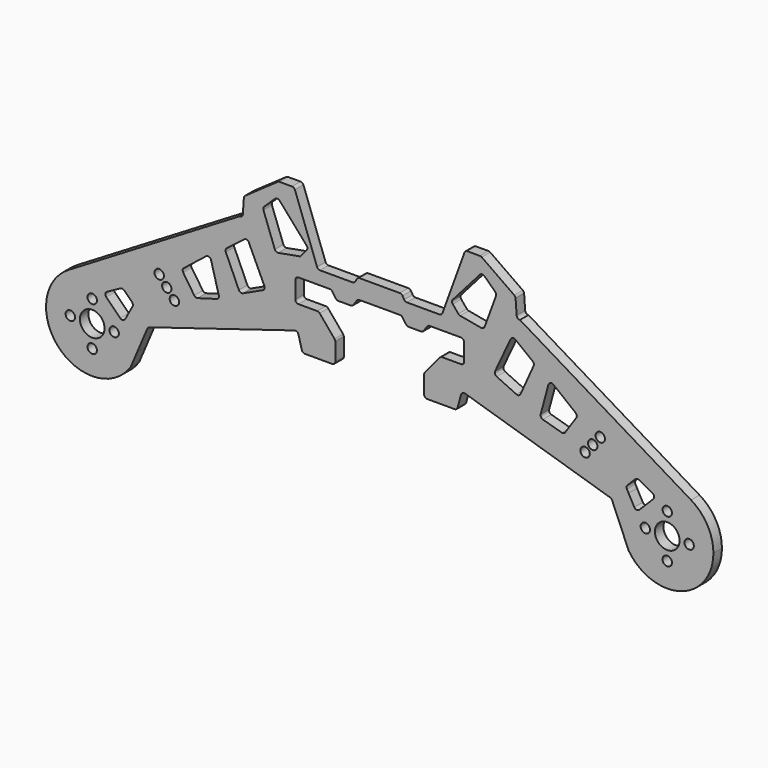
from build123d import *

# Parameters (mm, degrees)
F0_R     = 1.5
F0_R_2   = 3.9333333333
F1_DEPTH = 3.4


# Not quite as in the source:
# - a feature names something its author has since deleted; it is built from what else it names


with BuildPart() as f1:
    # F0 (on Front) → F1 (new body)
    with BuildSketch(Plane.XZ):
        with BuildLine():
            Line((-7.1178994687, 16.5873828769), (-61.7975655436, 49.4659744566))
            ThreePointArc((-61.7975655436, 49.4659744566), (-62.5109986563, 49.7167601817), (-62.8448613654, 50.3952997734))
            Line((-62.8448613654, 50.3952997734), (-63.1718740996, 55.0933258641))
            ThreePointArc((-63.1718740996, 55.0933258641), (-63.2990261516, 55.5161722641), (-63.5958839046, 55.8430395106))
            Line((-63.5958839046, 55.8430395106), (-74.0052830565, 63.131779265))
            ThreePointArc((-74.0052830565, 63.131779265), (-74.2781536934, 63.2663441715), (-74.5788594929, 63.3126272207))
            Line((-74.5788594929, 63.3126272207), (-78.5633531658, 63.3126272207))
            ThreePointArc((-78.5633531658, 63.3126272207), (-79.1369296021, 63.131779265), (-79.5030457866, 62.6546473641))
            Line((-79.5030457866, 62.6546473641), (-86.5485187746, 43.2973694201))
            ThreePointArc((-86.5485187746, 43.2973694201), (-86.914634959, 42.8202375192), (-87.4882113954, 42.6393895635))
            Line((-87.4882113954, 42.6393895635), (-97.9108611262, 42.6393895635))
            ThreePointArc((-97.9108611262, 42.6393895635), (-98.4108611262, 42.7733641597), (-98.77688653, 43.1393895635))
            Line((-98.77688653, 43.1393895635), (-99.2965017722, 44.0393895635))
            ThreePointArc((-99.2965017722, 44.0393895635), (-99.662527176, 44.4054149672), (-100.162527176, 44.5393895635))
            Line((-100.162527176, 44.5393895635), (-106.5851769068, 44.5393895635))
            Line((-106.5851769068, 44.5393895635), (-113.0078266377, 44.5393895635))
            ThreePointArc((-113.0078266377, 44.5393895635), (-113.5078266377, 44.4054149672), (-113.8738520414, 44.0393895635))
            Line((-113.8738520414, 44.0393895635), (-114.3934672837, 43.1393895635))
            ThreePointArc((-114.3934672837, 43.1393895635), (-114.7594926875, 42.7733641597), (-115.2594926875, 42.6393895635))
            Line((-115.2594926875, 42.6393895635), (-125.6821424183, 42.6393895635))
            ThreePointArc((-125.6821424183, 42.6393895635), (-126.2557188547, 42.8202375192), (-126.6218350391, 43.2973694201))
            Line((-126.6218350391, 43.2973694201), (-133.6673080271, 62.6546473641))
            ThreePointArc((-133.6673080271, 62.6546473641), (-134.0334242115, 63.131779265), (-134.6070006479, 63.3126272207))
            Line((-134.6070006479, 63.3126272207), (-138.5914943208, 63.3126272207))
            ThreePointArc((-138.5914943208, 63.3126272207), (-138.8922001203, 63.2663441715), (-139.1650707571, 63.131779265))
            Line((-139.1650707571, 63.131779265), (-149.5744699091, 55.8430395106))
            ThreePointArc((-149.5744699091, 55.8430395106), (-149.871327662, 55.5161722641), (-149.9984797141, 55.0933258641))
            Line((-149.9984797141, 55.0933258641), (-150.3254924483, 50.3952997734))
            ThreePointArc((-150.3254924483, 50.3952997734), (-150.6593551574, 49.7167601817), (-151.37278827, 49.4659744566))
            Line((-151.37278827, 49.4659744566), (-206.0524543449, 16.5873828769))
            ThreePointArc((-206.0524543449, 16.5873828769), (-198.1769936039, 18.6940314027), (-190.3854230638, 16.295640606))
            Line((-190.3854230638, 16.295640606), (-189.4141088114, 16.8207943138))
            ThreePointArc((-189.4141088114, 16.8207943138), (-188.794138811, 16.9306567145), (-188.2314016119, 16.6482396589))
            Line((-188.2314016119, 16.6482396589), (-185.7499602594, 14.1667983063))
            ThreePointArc((-185.7499602594, 14.1667983063), (-185.4675432037, 13.6040611073), (-185.5774056045, 12.9840911069))
            Line((-185.5774056045, 12.9840911069), (-186.1025593122, 12.0127768544))
            ThreePointArc((-186.1025593122, 12.0127768544), (-184.3145855529, 8.1545552233), (-183.7016118472, 3.9465880711))
            ThreePointArc((-183.7016118472, 3.9465880711), (-183.7928297697, 2.3087211638), (-184.0653553056, 0.6911122655))
            Line((-184.0653553056, 0.6911122655), (-180.8282501237, 8.3172541668))
            ThreePointArc((-180.8282501237, 8.3172541668), (-180.5768758766, 8.6696678638), (-180.200116975, 8.8828277943))
            Line((-180.200116975, 8.8828277943), (-133.8210939721, 23.0623181023))
            ThreePointArc((-133.8210939721, 23.0623181023), (-133.0439126471, 22.9806330535), (-132.5627964411, 22.3648323915))
            Line((-132.5627964411, 22.3648323915), (-131.4764959757, 18.3107038626))
            ThreePointArc((-131.4764959757, 18.3107038626), (-131.1193315785, 17.7761695674), (-130.5105701495, 17.5695229077))
            Line((-130.5105701495, 17.5695229077), (-121.7778971374, 17.5695229077))
            ThreePointArc((-121.7778971374, 17.5695229077), (-121.0707903562, 17.8624161265), (-120.7778971374, 18.5695229077))
            Line((-120.7778971374, 18.5695229077), (-120.7778971374, 24.2055526735))
            ThreePointArc((-120.7778971374, 24.2055526735), (-120.8382045166, 24.5475728168), (-121.0118526943, 24.8483402831))
            Line((-121.0118526943, 24.8483402831), (-125.7811581324, 30.5321771731))
            ThreePointArc((-125.7811581324, 30.5321771731), (-126.1245843138, 30.7956973505), (-126.5472025755, 30.8893895635))
            Line((-126.5472025755, 30.8893895635), (-132.5472025755, 30.8893895635))
            ThreePointArc((-132.5472025755, 30.8893895635), (-133.2543093567, 31.1822827823), (-133.5472025755, 31.8893895635))
            Line((-133.5472025755, 31.8893895635), (-133.5472025755, 37.3893895635))
            ThreePointArc((-133.5472025755, 37.3893895635), (-133.2543093567, 38.0964963446), (-132.5472025755, 38.3893895635))
            Line((-132.5472025755, 38.3893895635), (-122.5472025755, 38.3893895635))
            ThreePointArc((-122.5472025755, 38.3893895635), (-122.0854539623, 38.2764003966), (-121.7280505312, 37.9629659998))
            Line((-121.7280505312, 37.9629659998), (-120.6044912096, 36.3583569942))
            ThreePointArc((-120.6044912096, 36.3583569942), (-120.2470877786, 36.0449225974), (-119.7853391653, 35.9319334306))
            Line((-119.7853391653, 35.9319334306), (-115.8264732664, 35.9319334306))
            ThreePointArc((-115.8264732664, 35.9319334306), (-115.3647246532, 36.0449225974), (-115.0073212222, 36.3583569942))
            Line((-115.0073212222, 36.3583569942), (-113.8837619006, 37.9629659998))
            ThreePointArc((-113.8837619006, 37.9629659998), (-113.5263584695, 38.2764003966), (-113.0646098563, 38.3893895635))
            Line((-113.0646098563, 38.3893895635), (-106.5851769068, 38.3893895635))
            Line((-106.5851769068, 38.3893895635), (-100.1057439574, 38.3893895635))
            ThreePointArc((-100.1057439574, 38.3893895635), (-99.6439953442, 38.2764003966), (-99.2865919131, 37.9629659998))
            Line((-99.2865919131, 37.9629659998), (-98.1630325915, 36.3583569942))
            ThreePointArc((-98.1630325915, 36.3583569942), (-97.8056291605, 36.0449225974), (-97.3438805472, 35.9319334306))
            Line((-97.3438805472, 35.9319334306), (-93.3850146483, 35.9319334306))
            ThreePointArc((-93.3850146483, 35.9319334306), (-92.9232660351, 36.0449225974), (-92.5658626041, 36.3583569942))
            Line((-92.5658626041, 36.3583569942), (-91.4423032825, 37.9629659998))
            ThreePointArc((-91.4423032825, 37.9629659998), (-91.0848998514, 38.2764003966), (-90.6231512382, 38.3893895635))
            Line((-90.6231512382, 38.3893895635), (-80.6231512382, 38.3893895635))
            ThreePointArc((-80.6231512382, 38.3893895635), (-79.916044457, 38.0964963446), (-79.6231512382, 37.3893895635))
            Line((-79.6231512382, 37.3893895635), (-79.6231512382, 31.8893895635))
            ThreePointArc((-79.6231512382, 31.8893895635), (-79.916044457, 31.1822827823), (-80.6231512382, 30.8893895635))
            Line((-80.6231512382, 30.8893895635), (-86.6231512382, 30.8893895635))
            ThreePointArc((-86.6231512382, 30.8893895635), (-87.0457694999, 30.7956973505), (-87.3891956813, 30.5321771731))
            Line((-87.3891956813, 30.5321771731), (-92.1585011194, 24.8483402831))
            ThreePointArc((-92.1585011194, 24.8483402831), (-92.332149297, 24.5475728168), (-92.3924566763, 24.2055526735))
            Line((-92.3924566763, 24.2055526735), (-92.3924566763, 18.5695229077))
            ThreePointArc((-92.3924566763, 18.5695229077), (-92.0995634574, 17.8624161265), (-91.3924566763, 17.5695229077))
            Line((-91.3924566763, 17.5695229077), (-82.6597836642, 17.5695229077))
            ThreePointArc((-82.6597836642, 17.5695229077), (-82.0510222352, 17.7761695674), (-81.6938578379, 18.3107038626))
            Line((-81.6938578379, 18.3107038626), (-80.6075573726, 22.3648323915))
            ThreePointArc((-80.6075573726, 22.3648323915), (-80.1264411666, 22.9806330535), (-79.3492598416, 23.0623181023))
            Line((-79.3492598416, 23.0623181023), (-32.9702368387, 8.8828277943))
            ThreePointArc((-32.9702368387, 8.8828277943), (-32.5934779371, 8.6696678638), (-32.34210369, 8.3172541668))
            Line((-32.34210369, 8.3172541668), (-29.1049985081, 0.6911122655))
            ThreePointArc((-29.1049985081, 0.6911122655), (-29.2356014795, 6.5587308466), (-27.0677945015, 12.0127768544))
            Line((-27.0677945015, 12.0127768544), (-27.5929482092, 12.9840911069))
            ThreePointArc((-27.5929482092, 12.9840911069), (-27.70281061, 13.6040611073), (-27.4203935543, 14.1667983063))
            Line((-27.4203935543, 14.1667983063), (-24.9389522018, 16.6482396589))
            ThreePointArc((-24.9389522018, 16.6482396589), (-24.3762150027, 16.9306567145), (-23.7562450023, 16.8207943138))
            Line((-23.7562450023, 16.8207943138), (-22.7849307499, 16.295640606))
            ThreePointArc((-22.7849307499, 16.295640606), (-14.9933602098, 18.6940314027), (-7.1178994687, 16.5873828769))
        make_face()
        with Locations((-172.2004054547, 19.0294891768)):
            Circle(F0_R, mode=Mode.SUBTRACT)
        with Locations((-174.6239277514, 21.9184296078)):
            Circle(F0_R, mode=Mode.SUBTRACT)
        with Locations((-177.047450048, 24.8073700389)):
            Circle(F0_R, mode=Mode.SUBTRACT)
        with Locations((-40.969948359, 19.0294891768)):
            Circle(F0_R, mode=Mode.SUBTRACT)
        with Locations((-38.5464260623, 21.9184296078)):
            Circle(F0_R, mode=Mode.SUBTRACT)
        with Locations((-36.1229037657, 24.8073700389)):
            Circle(F0_R, mode=Mode.SUBTRACT)
        with BuildLine():
            Line((-158.6937889669, 23.8370476138), (-164.7364836334, 22.1040143276))
            ThreePointArc((-164.7364836334, 22.1040143276), (-165.3553883304, 22.1260077517), (-165.8426587786, 22.5082305205))
            Line((-165.8426587786, 22.5082305205), (-169.3786973616, 27.780185676))
            ThreePointArc((-169.3786973616, 27.780185676), (-169.5362483524, 28.4914029334), (-169.1694925986, 29.1208014707))
            Line((-169.1694925986, 29.1208014707), (-162.0717167673, 34.7484710934))
            ThreePointArc((-162.0717167673, 34.7484710934), (-161.1377185935, 34.9147353811), (-160.4851600582, 34.2261398829))
            Line((-160.4851600582, 34.2261398829), (-158.0042026399, 25.0595483909))
            ThreePointArc((-158.0042026399, 25.0595483909), (-158.0984856743, 24.3069906404), (-158.6937889669, 23.8370476138))
        make_face(mode=Mode.SUBTRACT)
        with BuildLine():
            Line((-155.4604981965, 39.1680426228), (-149.9236556169, 43.460411521))
            ThreePointArc((-149.9236556169, 43.460411521), (-149.075690405, 43.6420159728), (-148.4046588231, 43.0927056841))
            Line((-148.4046588231, 43.0927056841), (-143.4398764003, 32.4456954197))
            ThreePointArc((-143.4398764003, 32.4456954197), (-143.4064915666, 31.6810570146), (-143.9235659256, 31.1167693709))
            Line((-143.9235659256, 31.1167693709), (-150.2540395436, 28.1648210431))
            ThreePointArc((-150.2540395436, 28.1648210431), (-151.0257074463, 28.1340245947), (-151.5891952413, 28.662135642))
            Line((-151.5891952413, 28.662135642), (-155.7603466257, 37.968725336))
            ThreePointArc((-155.7603466257, 37.968725336), (-155.817948053, 38.6202686962), (-155.4604981965, 39.1680426228))
        make_face(mode=Mode.SUBTRACT)
        with BuildLine():
            Line((-129.9290728996, 46.9035901921), (-131.7075720486, 44.7654929954))
            ThreePointArc((-131.7075720486, 44.7654929954), (-131.972656186, 44.541115727), (-132.2984953392, 44.4209341783))
            Line((-132.2984953392, 44.4209341783), (-138.9870389565, 43.211949673))
            ThreePointArc((-138.9870389565, 43.211949673), (-139.6611905979, 43.3278404753), (-140.1031275449, 43.8499543026))
            Line((-140.1031275449, 43.8499543026), (-143.7391867896, 53.7081270257))
            ThreePointArc((-143.7391867896, 53.7081270257), (-143.7756511287, 54.2777769012), (-143.4945346139, 54.7745707555))
            Line((-143.4945346139, 54.7745707555), (-140.0367729145, 58.1035511138))
            ThreePointArc((-140.0367729145, 58.1035511138), (-139.3014635713, 58.3822846563), (-138.5919682195, 58.0431850192))
            Line((-138.5919682195, 58.0431850192), (-129.9466279079, 48.2031136398))
            ThreePointArc((-129.9466279079, 48.2031136398), (-129.6979595611, 47.5565925544), (-129.9290728996, 46.9035901921))
        make_face(mode=Mode.SUBTRACT)
        with BuildLine():
            ThreePointArc((-61.5811585724, 28.662135642), (-62.1446463673, 28.1340245947), (-62.9163142701, 28.1648210431))
            Line((-62.9163142701, 28.1648210431), (-69.2467878881, 31.1167693709))
            ThreePointArc((-69.2467878881, 31.1167693709), (-69.7638622471, 31.6810570146), (-69.7304774134, 32.4456954197))
            Line((-69.7304774134, 32.4456954197), (-64.7656949906, 43.0927056841))
            ThreePointArc((-64.7656949906, 43.0927056841), (-64.0946634086, 43.6420159728), (-63.2466981968, 43.460411521))
            Line((-63.2466981968, 43.460411521), (-57.7098556172, 39.1680426228))
            ThreePointArc((-57.7098556172, 39.1680426228), (-57.3524057607, 38.6202686962), (-57.410007188, 37.968725336))
            Line((-57.410007188, 37.968725336), (-61.5811585724, 28.662135642))
        make_face(mode=Mode.SUBTRACT)
        with BuildLine():
            Line((-43.791656452, 27.780185676), (-47.3276950351, 22.5082305205))
            ThreePointArc((-47.3276950351, 22.5082305205), (-47.8149654833, 22.1260077517), (-48.4338701803, 22.1040143276))
            Line((-48.4338701803, 22.1040143276), (-54.4765648468, 23.8370476138))
            ThreePointArc((-54.4765648468, 23.8370476138), (-55.0718681394, 24.3069906404), (-55.1661511738, 25.0595483909))
            Line((-55.1661511738, 25.0595483909), (-52.6851937555, 34.2261398829))
            ThreePointArc((-52.6851937555, 34.2261398829), (-52.0326352202, 34.9147353811), (-51.0986370464, 34.7484710934))
            Line((-51.0986370464, 34.7484710934), (-44.0008612151, 29.1208014707))
            ThreePointArc((-44.0008612151, 29.1208014707), (-43.6341054613, 28.4914029334), (-43.791656452, 27.780185676))
        make_face(mode=Mode.SUBTRACT)
        with BuildLine():
            Line((-83.2237259058, 48.2031136398), (-74.5783855942, 58.0431850192))
            ThreePointArc((-74.5783855942, 58.0431850192), (-73.8688902424, 58.3822846563), (-73.1335808991, 58.1035511138))
            Line((-73.1335808991, 58.1035511138), (-69.6758191998, 54.7745707555))
            ThreePointArc((-69.6758191998, 54.7745707555), (-69.394702685, 54.2777769012), (-69.4311670241, 53.7081270257))
            Line((-69.4311670241, 53.7081270257), (-73.0672262687, 43.8499543026))
            ThreePointArc((-73.0672262687, 43.8499543026), (-73.5091632157, 43.3278404753), (-74.1833148572, 43.211949673))
            Line((-74.1833148572, 43.211949673), (-80.8718584745, 44.4209341783))
            ThreePointArc((-80.8718584745, 44.4209341783), (-81.1976976277, 44.541115727), (-81.462781765, 44.7654929954))
            Line((-81.462781765, 44.7654929954), (-83.2412809141, 46.9035901921))
            ThreePointArc((-83.2412809141, 46.9035901921), (-83.4723942526, 47.5565925544), (-83.2237259058, 48.2031136398))
        make_face(mode=Mode.SUBTRACT)
        with BuildLine():
            ThreePointArc((0.0312580335, 3.9465880711), (-1.8798376744, 11.2077888381), (-7.1178994687, 16.5873828769))
            ThreePointArc((-7.1178994687, 16.5873828769), (-14.9933602098, 18.6940314027), (-22.7849307499, 16.295640606))
            Line((-22.7849307499, 16.295640606), (-19.4344655334, 14.4841679269))
            ThreePointArc((-19.4344655334, 14.4841679269), (-18.9205421148, 13.748876073), (-19.2029591705, 12.8973997096))
            Line((-19.2029591705, 12.8973997096), (-23.6695536051, 8.430805275))
            ThreePointArc((-23.6695536051, 8.430805275), (-24.5210299684, 8.1483882193), (-25.2563218223, 8.662311638))
            Line((-25.2563218223, 8.662311638), (-27.0677945015, 12.0127768544))
            ThreePointArc((-27.0677945015, 12.0127768544), (-29.2356014795, 6.5587308466), (-29.1049985081, 0.6911122655))
            Line((-29.1049985081, 0.6911122655), (-27.0540688086, -4.140575319))
            ThreePointArc((-27.0540688086, -4.140575319), (-10.4987639406, -10.1868575619), (0.0312580335, 3.9465880711))
        make_face()
        with Locations((-14.7187419665, -3.0534119289)):
            Circle(F0_R, mode=Mode.SUBTRACT)
        with Locations((-21.7187419665, 3.9465880711)):
            Circle(F0_R, mode=Mode.SUBTRACT)
        with Locations((-14.7187419665, 3.9465880711)):
            Circle(F0_R_2, mode=Mode.SUBTRACT)
        with Locations((-7.7187419665, 3.9465880711)):
            Circle(F0_R, mode=Mode.SUBTRACT)
        with Locations((-14.7187419665, 10.9465880711)):
            Circle(F0_R, mode=Mode.SUBTRACT)
        with BuildLine():
            ThreePointArc((-190.3854230638, 16.295640606), (-198.1769936039, 18.6940314027), (-206.0524543449, 16.5873828769))
            ThreePointArc((-206.0524543449, 16.5873828769), (-209.0825054242, -6.2782151914), (-186.116285005, -4.140575319))
            Line((-186.116285005, -4.140575319), (-184.0653553056, 0.6911122655))
            ThreePointArc((-184.0653553056, 0.6911122655), (-183.7928297697, 2.3087211638), (-183.7016118472, 3.9465880711))
            ThreePointArc((-183.7016118472, 3.9465880711), (-184.3145855529, 8.1545552233), (-186.1025593122, 12.0127768544))
            Line((-186.1025593122, 12.0127768544), (-187.9140319913, 8.662311638))
            ThreePointArc((-187.9140319913, 8.662311638), (-188.6493238453, 8.1483882193), (-189.5008002086, 8.430805275))
            Line((-189.5008002086, 8.430805275), (-193.9673946432, 12.8973997096))
            ThreePointArc((-193.9673946432, 12.8973997096), (-194.2498116989, 13.748876073), (-193.7358882803, 14.4841679269))
            Line((-193.7358882803, 14.4841679269), (-190.3854230638, 16.295640606))
        make_face()
        with Locations((-198.4516118472, -3.0534119289)):
            Circle(F0_R, mode=Mode.SUBTRACT)
        with Locations((-205.4516118472, 3.9465880711)):
            Circle(F0_R, mode=Mode.SUBTRACT)
        with Locations((-198.4516118472, 3.9465880711)):
            Circle(F0_R_2, mode=Mode.SUBTRACT)
        with Locations((-191.4516118472, 3.9465880711)):
            Circle(F0_R, mode=Mode.SUBTRACT)
        with Locations((-198.4516118472, 10.9465880711)):
            Circle(F0_R, mode=Mode.SUBTRACT)
    extrude(amount=F1_DEPTH)


solid = f1.part
